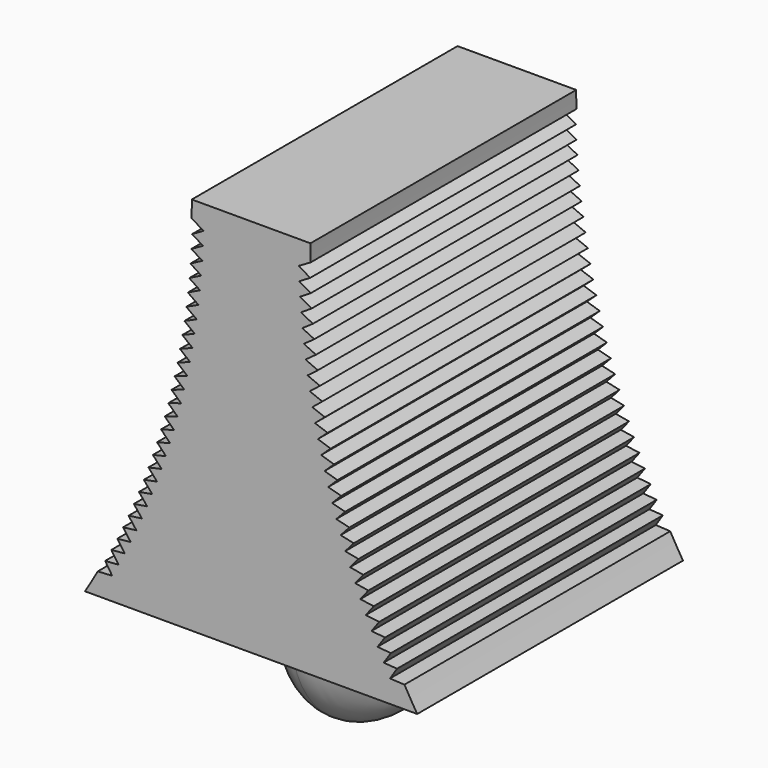
from build123d import *

# Parameters (mm, degrees)
F1_DEPTH = 14
F3_DEPTH = 1.25
F4_R     = 1.24999


# Not quite as in the source:
# - a fillet or chamfer is up to 0.001 mm smaller than in the source, because OpenCascade refuses the exact size


with BuildPart() as f1:
    # F0 (on Front) → F1 (new body)
    with BuildSketch(Plane.XZ):
        with BuildLine():
            Line((0, 8), (0, -8))
            Line((0, -8), (7, -8))
            ThreePointArc((7, -8), (6.7273087271, -7.5447627069), (6.462528291, -7.0848791956))
            Line((6.462528291, -7.0848791956), (5.8539806535, -7.0529865653))
            Line((5.8539806535, -7.0529865653), (6.1514320159, -6.5949516339))
            Line((6.1514320159, -6.5949516339), (5.5856572031, -6.5550071363))
            Line((5.5856572031, -6.5550071363), (5.8913609435, -6.1024383189))
            Line((5.8913609435, -6.1024383189), (5.326402994, -6.0522465166))
            Line((5.326402994, -6.0522465166), (5.6402586914, -5.605292478))
            Line((5.6402586914, -5.605292478), (5.0763031889, -5.5448698584))
            Line((5.0763031889, -5.5448698584), (5.3982077445, -5.1036774191))
            Line((5.3982077445, -5.1036774191), (4.8354399434, -5.0330438306))
            Line((4.8354399434, -5.0330438306), (5.1652876144, -4.5977579185))
            Line((5.1652876144, -4.5977579185), (4.603892379, -4.5169365636))
            Line((4.603892379, -4.5169365636), (4.9415748133, -4.087700166))
            Line((4.9415748133, -4.087700166), (4.3817365569, -3.9967175939))
            Line((4.3817365569, -3.9967175939), (4.7271428288, -3.5736717114))
            Line((4.7271428288, -3.5736717114), (4.1690454534, -3.4725578088))
            Line((4.1690454534, -3.4725578088), (4.5220621001, -3.0558414082))
            Line((4.5220621001, -3.0558414082), (3.9658889357, -2.9446293904))
            Line((3.9658889357, -2.9446293904), (4.3263999942, -2.5343793592))
            Line((4.3263999942, -2.5343793592), (3.7723337388, -2.4131057583))
            Line((3.7723337388, -2.4131057583), (4.1402207845, -2.0094568602))
            Line((4.1402207845, -2.0094568602), (3.5884434439, -1.8781615134))
            Line((3.5884434439, -1.8781615134), (3.9635856292, -1.4812463433))
            Line((3.9635856292, -1.4812463433), (3.4142784574, -1.3399723801))
            Line((3.4142784574, -1.3399723801), (3.7965525514, -0.9499213213))
            Line((3.7965525514, -0.9499213213), (3.2498959909, -0.7987151488))
            Line((3.2498959909, -0.7987151488), (3.6391764199, -0.4156563295))
            Line((3.6391764199, -0.4156563295), (3.0953500426, -0.2545676177))
            Line((3.0953500426, -0.2545676177), (3.4915089314, 0.1213731306))
            Line((3.4915089314, 0.1213731306), (2.9506913795, 0.2922914656))
            Line((2.9506913795, 0.2922914656), (3.3535985934, 0.6609906496))
            Line((3.3535985934, 0.6609906496), (2.8159675207, 0.8416824626))
            Line((2.8159675207, 0.8416824626), (3.2254907083, 1.203018968))
            Line((3.2254907083, 1.203018968), (2.6912227217, 1.3934249033))
            Line((2.6912227217, 1.3934249033), (3.1072273582, 1.7472800342))
            Line((3.1072273582, 1.7472800342), (2.5764979601, 1.9473375451))
            Line((2.5764979601, 1.9473375451), (2.9988473918, 2.2935950634))
            Line((2.9988473918, 2.2935950634), (2.4718309221, 2.5032384328))
            Line((2.4718309221, 2.5032384328), (2.9003864108, 2.8417845957))
            Line((2.9003864108, 2.8417845957), (2.3772559897, 3.0609449576))
            Line((2.3772559897, 3.0609449576), (2.8118767588, 3.3916685559))
            Line((2.8118767588, 3.3916685559), (2.2928042301, 3.6202739181))
            Line((2.2928042301, 3.6202739181), (2.7333475104, 3.9430663119))
            Line((2.7333475104, 3.9430663119), (2.2185033848, 4.1810415796))
            Line((2.2185033848, 4.1810415796), (2.6648244619, 4.4957967344))
            Line((2.6648244619, 4.4957967344), (2.1543778611, 4.7430637348))
            Line((2.1543778611, 4.7430637348), (2.6063301224, 5.0496782564))
            Line((2.6063301224, 5.0496782564), (2.1004487236, 5.3061557644))
            Line((2.1004487236, 5.3061557644), (2.5578837068, 5.6045289327))
            Line((2.5578837068, 5.6045289327), (2.0567336876, 5.8701326978))
            Line((2.0567336876, 5.8701326978), (2.5195011293, 6.1601664998))
            Line((2.5195011293, 6.1601664998), (2.0232471131, 6.4348092734))
            Line((2.0232471131, 6.4348092734), (2.4911949982, 6.7164084356))
            Line((2.4911949982, 6.7164084356), (2, 7))
            Line((2, 7), (2.5081348332, 7.2933717827))
            ThreePointArc((2.5081348332, 7.2933717827), (2.5020337704, 7.6466624796), (2.5, 8))
            Line((2.5, 8), (0, 8))
        make_face()
        with BuildLine():
            ThreePointArc((-6.462528291, -7.0848791956), (-6.7273087271, -7.5447627069), (-7, -8))
            Line((-7, -8), (0, -8))
            Line((0, -8), (0, 8))
            Line((0, 8), (-2.5, 8))
            ThreePointArc((-2.5, 8), (-2.5020337704, 7.6466624796), (-2.5081348332, 7.2933717827))
            Line((-2.5081348332, 7.2933717827), (-2, 7))
            Line((-2, 7), (-2.4911949982, 6.7164084356))
            Line((-2.4911949982, 6.7164084356), (-2.0232471131, 6.4348092734))
            Line((-2.0232471131, 6.4348092734), (-2.5195011293, 6.1601664998))
            Line((-2.5195011293, 6.1601664998), (-2.0567336876, 5.8701326978))
            Line((-2.0567336876, 5.8701326978), (-2.5578837068, 5.6045289327))
            Line((-2.5578837068, 5.6045289327), (-2.1004487236, 5.3061557644))
            Line((-2.1004487236, 5.3061557644), (-2.6063301224, 5.0496782564))
            Line((-2.6063301224, 5.0496782564), (-2.1543778611, 4.7430637348))
            Line((-2.1543778611, 4.7430637348), (-2.6648244619, 4.4957967344))
            Line((-2.6648244619, 4.4957967344), (-2.2185033848, 4.1810415796))
            Line((-2.2185033848, 4.1810415796), (-2.7333475104, 3.9430663119))
            Line((-2.7333475104, 3.9430663119), (-2.2928042301, 3.6202739181))
            Line((-2.2928042301, 3.6202739181), (-2.8118767588, 3.3916685559))
            Line((-2.8118767588, 3.3916685559), (-2.3772559897, 3.0609449576))
            Line((-2.3772559897, 3.0609449576), (-2.9003864108, 2.8417845957))
            Line((-2.9003864108, 2.8417845957), (-2.4718309221, 2.5032384328))
            Line((-2.4718309221, 2.5032384328), (-2.9988473918, 2.2935950634))
            Line((-2.9988473918, 2.2935950634), (-2.5764979601, 1.9473375451))
            Line((-2.5764979601, 1.9473375451), (-3.1072273582, 1.7472800342))
            Line((-3.1072273582, 1.7472800342), (-2.6912227217, 1.3934249033))
            Line((-2.6912227217, 1.3934249033), (-3.2254907083, 1.203018968))
            Line((-3.2254907083, 1.203018968), (-2.8159675207, 0.8416824626))
            Line((-2.8159675207, 0.8416824626), (-3.3535985934, 0.6609906496))
            Line((-3.3535985934, 0.6609906496), (-2.9506913795, 0.2922914656))
            Line((-2.9506913795, 0.2922914656), (-3.4915089314, 0.1213731306))
            Line((-3.4915089314, 0.1213731306), (-3.0953500426, -0.2545676177))
            Line((-3.0953500426, -0.2545676177), (-3.6391764199, -0.4156563295))
            Line((-3.6391764199, -0.4156563295), (-3.2498959909, -0.7987151488))
            Line((-3.2498959909, -0.7987151488), (-3.7965525514, -0.9499213213))
            Line((-3.7965525514, -0.9499213213), (-3.4142784574, -1.3399723801))
            Line((-3.4142784574, -1.3399723801), (-3.9635856292, -1.4812463433))
            Line((-3.9635856292, -1.4812463433), (-3.5884434439, -1.8781615134))
            Line((-3.5884434439, -1.8781615134), (-4.1402207845, -2.0094568602))
            Line((-4.1402207845, -2.0094568602), (-3.7723337388, -2.4131057583))
            Line((-3.7723337388, -2.4131057583), (-4.3263999942, -2.5343793592))
            Line((-4.3263999942, -2.5343793592), (-3.9658889357, -2.9446293904))
            Line((-3.9658889357, -2.9446293904), (-4.5220621001, -3.0558414082))
            Line((-4.5220621001, -3.0558414082), (-4.1690454534, -3.4725578088))
            Line((-4.1690454534, -3.4725578088), (-4.7271428288, -3.5736717114))
            Line((-4.7271428288, -3.5736717114), (-4.3817365569, -3.9967175939))
            Line((-4.3817365569, -3.9967175939), (-4.9415748133, -4.087700166))
            Line((-4.9415748133, -4.087700166), (-4.603892379, -4.5169365636))
            Line((-4.603892379, -4.5169365636), (-5.1652876144, -4.5977579185))
            Line((-5.1652876144, -4.5977579185), (-4.8354399434, -5.0330438306))
            Line((-4.8354399434, -5.0330438306), (-5.3982077445, -5.1036774191))
            Line((-5.3982077445, -5.1036774191), (-5.0763031889, -5.5448698584))
            Line((-5.0763031889, -5.5448698584), (-5.6402586914, -5.605292478))
            Line((-5.6402586914, -5.605292478), (-5.326402994, -6.0522465166))
            Line((-5.326402994, -6.0522465166), (-5.8913609435, -6.1024383189))
            Line((-5.8913609435, -6.1024383189), (-5.5856572031, -6.5550071363))
            Line((-5.5856572031, -6.5550071363), (-6.1514320159, -6.5949516339))
            Line((-6.1514320159, -6.5949516339), (-5.8539806535, -7.0529865653))
            Line((-5.8539806535, -7.0529865653), (-6.462528291, -7.0848791956))
        make_face()
    extrude(amount=F1_DEPTH)

    # F2 (on Right) → F3 (join, symmetric)
    with BuildSketch(Plane.YZ):
        with BuildLine():
            Line((-9.4047106404, -8), (-11.9047106404, -8))
            ThreePointArc((-11.9047106404, -8), (-6.9047106404, -13), (-1.9047106404, -8))
            Line((-1.9047106404, -8), (-4.4047106404, -8))
            ThreePointArc((-4.4047106404, -8), (-6.9047106404, -10.5), (-9.4047106404, -8))
        make_face()
    extrude(amount=F3_DEPTH, both=True)

    # F4 (radius 1.25 in the source; OpenCascade refuses exactly that, so slightly less here)
    f4_edges = [f1.edges().sort_by_distance(p)[0] for p in [
        (1.25, -6.904711, -13),
        (-1.25, -6.904711, -13),
        (1.25, -6.904711, -10.5),
        (-1.25, -6.904711, -10.5),
    ]]
    fillet(f4_edges, radius=F4_R)


solid = f1.part
